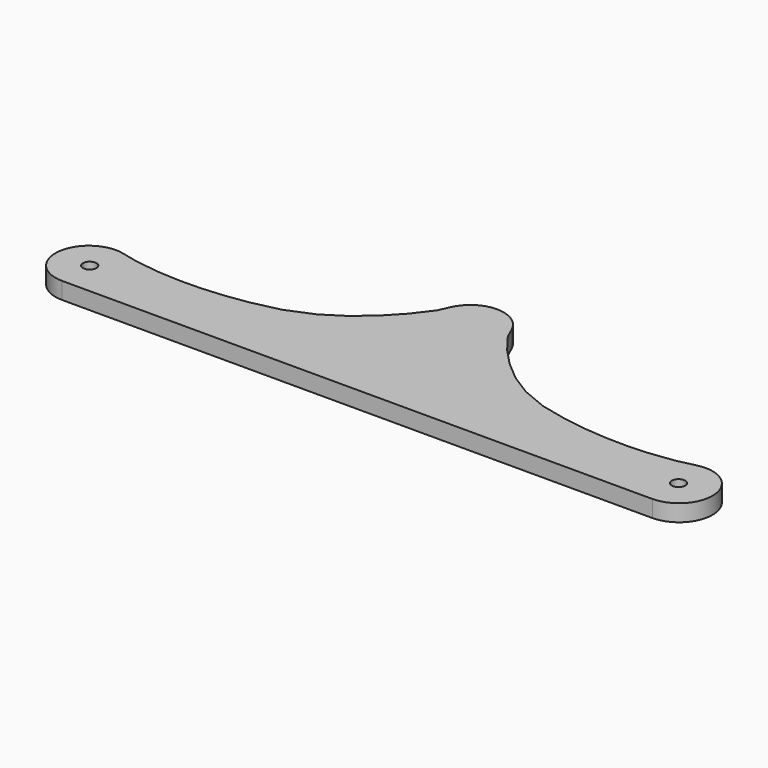
from build123d import *

# Parameters (mm, degrees)
F0_R     = 2
F1_DEPTH = 5


# Not quite as in the source:
# - ends of sketch curves that miss each other by under 0.0002 mm in the source are joined


with BuildPart() as f1:
    # F0 (on Top) → F1 (new body)
    with BuildSketch(Plane.XY):
        with BuildLine():
            ThreePointArc((-86.9239089763, -96.6023878966), (-99.0303580955, -105.1836331247), (-89.144034, -116.25))
            Line((-89.144034, -116.25), (86.235345, -116.25))
            ThreePointArc((86.235345, -116.25), (96.1216690408, -105.1836326404), (84.0152190261, -96.6023881141))
            Line((84.0152190261, -96.6023881141), (78.54514, -97.854584))
            Line((78.54514, -97.854584), (71.133383, -98.793694))
            Line((71.133383, -98.793694), (64.939287, -99.095039))
            Line((64.939287, -99.095039), (58.739872, -98.995936))
            Line((58.739872, -98.995936), (52.07042, -98.463421))
            Line((52.07042, -98.463421), (45.452353, -97.494386))
            Line((45.452353, -97.494386), (37.288225, -95.647643))
            Line((37.288225, -95.647643), (29.552302, -92.435031))
            Line((29.552302, -92.435031), (23.41918, -88.534685))
            Line((23.41918, -88.534685), (17.86875, -83.821678))
            Line((17.86875, -83.821678), (13.197325, -78.879824))
            Line((13.197325, -78.879824), (9.083287, -73.477642))
            Line((9.083287, -73.477642), (7.586324, -70.18701))
            ThreePointArc((7.586324, -70.18701), (-1.454345, -64.321401), (-10.4950136906, -70.1870101381))
            Line((-10.4950136906, -70.1870101381), (-11.991976, -73.477642))
            Line((-11.991976, -73.477642), (-16.106015, -78.879824))
            Line((-16.106015, -78.879824), (-20.77744, -83.821678))
            Line((-20.77744, -83.821678), (-26.32787, -88.534685))
            Line((-26.32787, -88.534685), (-32.460992, -92.435031))
            Line((-32.460992, -92.435031), (-40.196915, -95.647643))
            Line((-40.196915, -95.647643), (-48.361042, -97.494386))
            Line((-48.361042, -97.494386), (-54.979109, -98.463421))
            Line((-54.979109, -98.463421), (-61.648561, -98.995936))
            Line((-61.648561, -98.995936), (-67.847977, -99.095039))
            Line((-67.847977, -99.095039), (-74.042073, -98.793694))
            Line((-74.042073, -98.793694), (-81.45383, -97.854584))
            Line((-81.45383, -97.854584), (-86.9239089763, -96.6023878966))
        make_face()
        with Locations((-88.954345, -106.25)):
            Circle(F0_R, mode=Mode.SUBTRACT)
        with Locations((86.045655, -106.25)):
            Circle(F0_R, mode=Mode.SUBTRACT)
    extrude(amount=F1_DEPTH)


solid = f1.part
